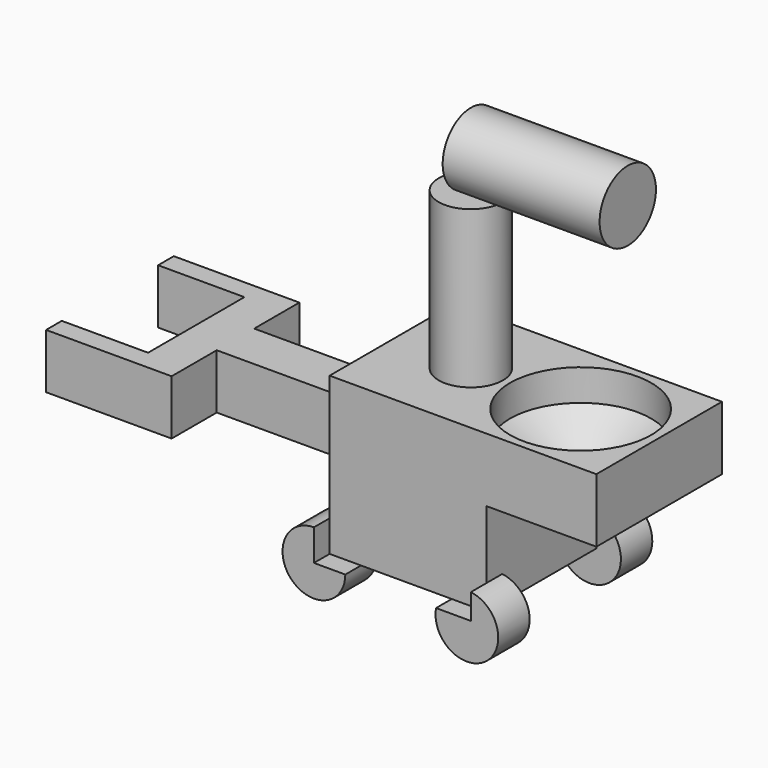
from build123d import *

# Parameters (mm, degrees)
F0_W      = 25.4
F0_H      = 25.4
F1_DEPTH  = 12.7
F3_DEPTH  = 3.175
F5_DEPTH  = 3.175
F6_R      = 5.2164072596
F7_DEPTH  = 25.4
F8_R      = 5.6995289673
F9_DEPTH  = 25.4
F12_W     = 7.5837243348
F12_H     = 8.8812420145
F13_DEPTH = 25.4
F14_W     = 5.954047665
F14_H     = 8.8812420145
F14_W_2   = 7.5837243348
F15_DEPTH = 6.35
F16_W     = 6.35
F16_H     = 8.8812420145
F16_W_2   = 13.97
F17_DEPTH = 3.175
F18_W     = 13.97
F18_H     = 8.8812420145
F18_W_2   = 6.35
F19_DEPTH = 3.175
F20_W     = 25.4
F20_H     = 10.3356431233
F21_DEPTH = 17.78
F23_D     = 22.86
F23_DEPTH = 5.08
F23_TIP   = 6.8678368755


# Not quite as in the source:
# - the program builds the solid bodies; features that only make, move or delete a surface that nothing else refers to are left out


with BuildPart() as f1:
    # F0 (on Front) → F1 (new body, symmetric)
    with BuildSketch(Plane.XZ):
        Rectangle(F0_W, F0_H)
    extrude(amount=F1_DEPTH, both=True)

    # F2 (on face) → F3 (join, symmetric)
    with BuildSketch(Plane.XZ.offset(12.7)):
        with BuildLine():
            ThreePointArc((-12.7, -7.62), (-16.2921024484, -16.2921024484), (-7.62, -12.7))
            Line((-7.62, -12.7), (-12.7, -12.7))
            Line((-12.7, -12.7), (-12.7, -7.62))
        make_face()
        with BuildLine():
            Line((12.7, -12.7), (7.0624674123, -12.7))
            ThreePointArc((7.0624674123, -12.7), (11.5896136049, -18.6885230146), (17.136607753, -13.6300334707))
            ThreePointArc((17.136607753, -13.6300334707), (15.8694041425, -10.2731027754), (12.7, -8.5909416461))
            Line((12.7, -8.5909416461), (12.7, -12.7))
        make_face()
    extrude(amount=F3_DEPTH, both=True)

    # F4 (on face) → F5 (join, symmetric)
    with BuildSketch(Plane(origin=(0, 12.7, 0), x_dir=(-1, 0, 0), z_dir=(0, 1, 0))):
        with BuildLine():
            ThreePointArc((-12.7, -7.9712862466), (-14.7674220428, -16.8935743083), (-6.5113730115, -12.9288407043))
            ThreePointArc((-6.5113730115, -12.9288407043), (-6.5126624138, -12.8143913027), (-6.5165299664, -12.7))
            Line((-6.5165299664, -12.7), (-12.7, -12.7))
            Line((-12.7, -12.7), (-12.7, -7.9712862466))
        make_face()
        with BuildLine():
            Line((12.7, -12.7), (6.8250320748, -12.7))
            ThreePointArc((6.8250320748, -12.7), (12.3480368398, -16.6116586986), (16.856369065, -11.5639269352))
            ThreePointArc((16.856369065, -11.5639269352), (15.6813943626, -8.314745896), (12.7, -6.568598528))
            Line((12.7, -6.568598528), (12.7, -12.7))
        make_face()
    extrude(amount=F5_DEPTH, both=True)

    # F6 (on face) → F7 (join)
    with BuildSketch(Plane.XY.offset(12.7)):
        Circle(F6_R)
    extrude(amount=F7_DEPTH)

    # F12 (on face) → F13 (join)
    with BuildSketch(Plane(origin=(-12.7, 0, 0), x_dir=(0, -1, 0), z_dir=(-1, 0, 0))):
        Rectangle(F12_W, F12_H)
    extrude(amount=F13_DEPTH)

    # F14 (on face) → F15 (join)
    with BuildSketch(Plane(origin=(-38.1, 0, 0), x_dir=(0, -1, 0), z_dir=(-1, 0, 0))):
        with Locations((-6.7688859999, 0)):
            Rectangle(F14_W, F14_H)
        Rectangle(F14_W_2, F14_H)
        with Locations((6.7688859999, 0)):
            Rectangle(F14_W, F14_H)
    extrude(amount=F15_DEPTH)

    # F16 (on face) → F17 (join)
    with BuildSketch(Plane(origin=(0, 9.7459098324, 0), x_dir=(-1, 0, 0), z_dir=(0, 1, 0))):
        with Locations((41.275, 0)):
            Rectangle(F16_W, F16_H)
        with Locations((51.435, 0)):
            Rectangle(F16_W_2, F16_H)
    extrude(amount=F17_DEPTH)

    # F18 (on face) → F19 (join)
    with BuildSketch(Plane.XZ.offset(9.7459098324)):
        with Locations((-51.435, 0)):
            Rectangle(F18_W, F18_H)
        with Locations((-41.275, 0)):
            Rectangle(F18_W_2, F18_H)
    extrude(amount=F19_DEPTH)

    # F20 (on face) → F21 (join)
    with BuildSketch(Plane.YZ.offset(12.7)):
        with Locations((0, 7.5321784383)):
            Rectangle(F20_W, F20_H)
    extrude(amount=F21_DEPTH)

    # F23
    with Locations(Plane.XY.offset(12.7)):
        with Locations((17.7709162235, 0)):
            Hole(F23_D / 2, depth=F23_DEPTH)
            with Locations((0, 0, -(F23_DEPTH + F23_TIP / 2))):  # 118° drill point
                Cone(0, F23_D / 2, F23_TIP, mode=Mode.SUBTRACT)


with BuildPart() as f9:
    # F8 (on Right) → F9 (new body)
    with BuildSketch(Plane.YZ):
        with Locations((0, 44.1520959139)):
            Circle(F8_R)
    extrude(amount=F9_DEPTH)


solid = Compound([f1.part, f9.part])
